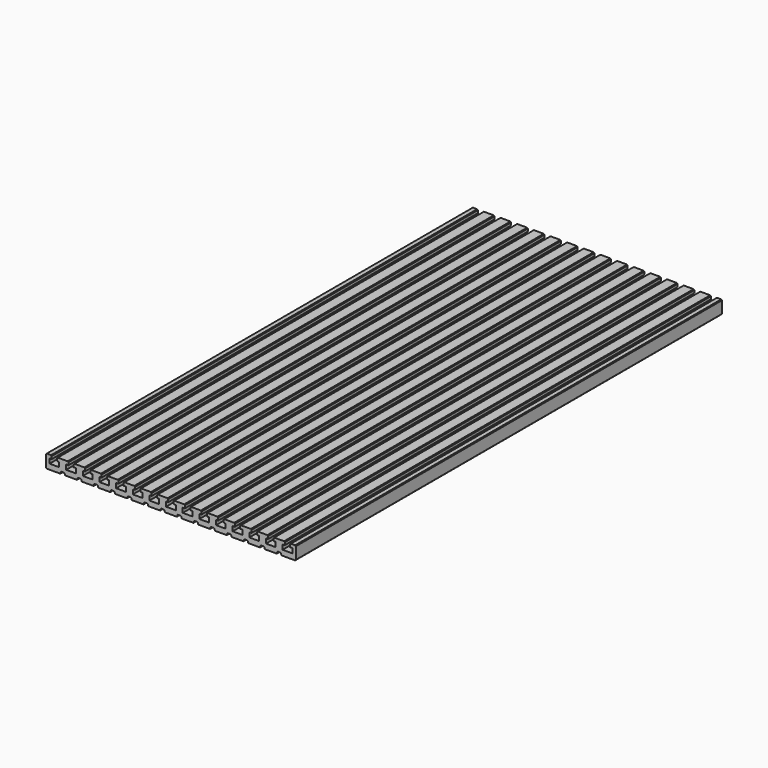
from build123d import *

# Parameters (mm, degrees)
F1_DEPTH = 800


# Not quite as in the source:
# - ends of sketch curves that miss each other by under 0.0002 mm in the source are joined


with BuildPart() as f1:
    # F0 (on Front) → F1 (new body)
    with BuildSketch(Plane.XZ):
        with BuildLine():
            Line((-187.5, -9), (-186.5, -10))
            Line((-186.5, -10), (-166.040705, -10))
            ThreePointArc((-166.040705, -10), (-165.9393586848, -9.787513692), (-165.8725056652, -9.5617878587))
            Line((-165.8725056652, -9.5617878587), (-165.527495, -7.938212))
            ThreePointArc((-165.527495, -7.938212), (-165.0042691575, -7.0843066242), (-164.060257, -6.75))
            Line((-164.060257, -6.75), (-160.939744, -6.75))
            ThreePointArc((-160.939744, -6.75), (-159.9957317617, -7.0843066896), (-159.4725056652, -7.9382121413))
            Line((-159.4725056652, -7.9382121413), (-159.127495, -9.561788))
            ThreePointArc((-159.127495, -9.561788), (-159.0606421883, -9.7875140224), (-158.9592950793, -10.0000000458))
            Line((-158.9592950793, -10.0000000458), (-141.040705, -10))
            ThreePointArc((-141.040705, -10), (-140.9393586848, -9.787513692), (-140.8725056652, -9.5617878587))
            Line((-140.8725056652, -9.5617878587), (-140.527495, -7.938212))
            ThreePointArc((-140.527495, -7.938212), (-140.0042691575, -7.0843066242), (-139.060257, -6.75))
            Line((-139.060257, -6.75), (-135.939744, -6.75))
            ThreePointArc((-135.939744, -6.75), (-134.9957317617, -7.0843066896), (-134.4725056652, -7.9382121413))
            Line((-134.4725056652, -7.9382121413), (-134.127495, -9.561788))
            ThreePointArc((-134.127495, -9.561788), (-134.0606421883, -9.7875140224), (-133.9592950793, -10.0000000458))
            Line((-133.9592950793, -10.0000000458), (-116.040705, -10))
            ThreePointArc((-116.040705, -10), (-115.9393586848, -9.787513692), (-115.8725056652, -9.5617878587))
            Line((-115.8725056652, -9.5617878587), (-115.527495, -7.938212))
            ThreePointArc((-115.527495, -7.938212), (-115.0042691575, -7.0843066242), (-114.060257, -6.75))
            Line((-114.060257, -6.75), (-110.939744, -6.75))
            ThreePointArc((-110.939744, -6.75), (-109.9957317617, -7.0843066896), (-109.4725056652, -7.9382121413))
            Line((-109.4725056652, -7.9382121413), (-109.127495, -9.561788))
            ThreePointArc((-109.127495, -9.561788), (-109.0606421883, -9.7875140224), (-108.9592950793, -10.0000000458))
            Line((-108.9592950793, -10.0000000458), (-91.040705, -10))
            ThreePointArc((-91.040705, -10), (-90.9393586848, -9.787513692), (-90.8725056652, -9.5617878587))
            Line((-90.8725056652, -9.5617878587), (-90.527495, -7.938212))
            ThreePointArc((-90.527495, -7.938212), (-90.0042691575, -7.0843066242), (-89.060257, -6.75))
            Line((-89.060257, -6.75), (-85.939744, -6.75))
            ThreePointArc((-85.939744, -6.75), (-84.9957317617, -7.0843066896), (-84.4725056652, -7.9382121413))
            Line((-84.4725056652, -7.9382121413), (-84.127495, -9.561788))
            ThreePointArc((-84.127495, -9.561788), (-84.0606421883, -9.7875140224), (-83.9592950793, -10.0000000458))
            Line((-83.9592950793, -10.0000000458), (-66.040705, -10))
            ThreePointArc((-66.040705, -10), (-65.9393586848, -9.787513692), (-65.8725056652, -9.5617878587))
            Line((-65.8725056652, -9.5617878587), (-65.527495, -7.938212))
            ThreePointArc((-65.527495, -7.938212), (-65.0042691575, -7.0843066242), (-64.060257, -6.75))
            Line((-64.060257, -6.75), (-60.939744, -6.75))
            ThreePointArc((-60.939744, -6.75), (-59.9957317617, -7.0843066896), (-59.4725056652, -7.9382121413))
            Line((-59.4725056652, -7.9382121413), (-59.127495, -9.561788))
            ThreePointArc((-59.127495, -9.561788), (-59.0606421883, -9.7875140224), (-58.9592950793, -10.0000000458))
            Line((-58.9592950793, -10.0000000458), (-41.040705, -10))
            ThreePointArc((-41.040705, -10), (-40.9393586848, -9.787513692), (-40.8725056652, -9.5617878587))
            Line((-40.8725056652, -9.5617878587), (-40.527495, -7.938212))
            ThreePointArc((-40.527495, -7.938212), (-40.0042691575, -7.0843066242), (-39.060257, -6.75))
            Line((-39.060257, -6.75), (-35.939744, -6.75))
            ThreePointArc((-35.939744, -6.75), (-34.9957317617, -7.0843066896), (-34.4725056652, -7.9382121413))
            Line((-34.4725056652, -7.9382121413), (-34.127495, -9.561788))
            ThreePointArc((-34.127495, -9.561788), (-34.0606421883, -9.7875140224), (-33.9592950793, -10.0000000458))
            Line((-33.9592950793, -10.0000000458), (-16.040705, -10))
            ThreePointArc((-16.040705, -10), (-15.9393586848, -9.787513692), (-15.8725056652, -9.5617878587))
            Line((-15.8725056652, -9.5617878587), (-15.527495, -7.938212))
            ThreePointArc((-15.527495, -7.938212), (-15.0042691575, -7.0843066242), (-14.060257, -6.75))
            Line((-14.060257, -6.75), (-10.939744, -6.75))
            ThreePointArc((-10.939744, -6.75), (-9.9957317617, -7.0843066896), (-9.4725056652, -7.9382121413))
            Line((-9.4725056652, -7.9382121413), (-9.127495, -9.561788))
            ThreePointArc((-9.127495, -9.561788), (-9.0606421883, -9.7875140224), (-8.9592950793, -10.0000000458))
            Line((-8.9592950793, -10.0000000458), (8.959295, -10))
            ThreePointArc((8.959295, -10), (9.0606413152, -9.787513692), (9.1274943348, -9.5617878587))
            Line((9.1274943348, -9.5617878587), (9.472505, -7.938212))
            ThreePointArc((9.472505, -7.938212), (9.9957308425, -7.0843066242), (10.939743, -6.75))
            Line((10.939743, -6.75), (14.060256, -6.75))
            ThreePointArc((14.060256, -6.75), (15.0042682383, -7.0843066896), (15.5274943348, -7.9382121413))
            Line((15.5274943348, -7.9382121413), (15.872505, -9.561788))
            ThreePointArc((15.872505, -9.561788), (15.9393578117, -9.7875140224), (16.0407049207, -10.0000000458))
            Line((16.0407049207, -10.0000000458), (33.959295, -10))
            ThreePointArc((33.959295, -10), (34.0606413152, -9.787513692), (34.1274943348, -9.5617878587))
            Line((34.1274943348, -9.5617878587), (34.472505, -7.938212))
            ThreePointArc((34.472505, -7.938212), (34.9957308425, -7.0843066242), (35.939743, -6.75))
            Line((35.939743, -6.75), (39.060256, -6.75))
            ThreePointArc((39.060256, -6.75), (40.0042682383, -7.0843066896), (40.5274943348, -7.9382121413))
            Line((40.5274943348, -7.9382121413), (40.872505, -9.561788))
            ThreePointArc((40.872505, -9.561788), (40.9393578117, -9.7875140224), (41.0407049207, -10.0000000458))
            Line((41.0407049207, -10.0000000458), (58.959295, -10))
            ThreePointArc((58.959295, -10), (59.0606413152, -9.787513692), (59.1274943348, -9.5617878587))
            Line((59.1274943348, -9.5617878587), (59.472505, -7.938212))
            ThreePointArc((59.472505, -7.938212), (59.9957308425, -7.0843066242), (60.939743, -6.75))
            Line((60.939743, -6.75), (64.060256, -6.75))
            ThreePointArc((64.060256, -6.75), (65.0042682383, -7.0843066896), (65.5274943348, -7.9382121413))
            Line((65.5274943348, -7.9382121413), (65.872505, -9.561788))
            ThreePointArc((65.872505, -9.561788), (65.9393578117, -9.7875140224), (66.0407049207, -10.0000000458))
            Line((66.0407049207, -10.0000000458), (83.959295, -10))
            ThreePointArc((83.959295, -10), (84.0606413152, -9.787513692), (84.1274943348, -9.5617878587))
            Line((84.1274943348, -9.5617878587), (84.472505, -7.938212))
            ThreePointArc((84.472505, -7.938212), (84.9957308425, -7.0843066242), (85.939743, -6.75))
            Line((85.939743, -6.75), (89.060256, -6.75))
            ThreePointArc((89.060256, -6.75), (90.0042682383, -7.0843066896), (90.5274943348, -7.9382121413))
            Line((90.5274943348, -7.9382121413), (90.872505, -9.561788))
            ThreePointArc((90.872505, -9.561788), (90.9393578117, -9.7875140224), (91.0407049207, -10.0000000458))
            Line((91.0407049207, -10.0000000458), (108.959295, -10))
            ThreePointArc((108.959295, -10), (109.0606413152, -9.787513692), (109.1274943348, -9.5617878587))
            Line((109.1274943348, -9.5617878587), (109.472505, -7.938212))
            ThreePointArc((109.472505, -7.938212), (109.9957308425, -7.0843066242), (110.939743, -6.75))
            Line((110.939743, -6.75), (114.060256, -6.75))
            ThreePointArc((114.060256, -6.75), (115.0042682383, -7.0843066896), (115.5274943348, -7.9382121413))
            Line((115.5274943348, -7.9382121413), (115.872505, -9.561788))
            ThreePointArc((115.872505, -9.561788), (115.9393578117, -9.7875140224), (116.0407049207, -10.0000000458))
            Line((116.0407049207, -10.0000000458), (133.959295, -10))
            ThreePointArc((133.959295, -10), (134.0606413152, -9.787513692), (134.1274943348, -9.5617878587))
            Line((134.1274943348, -9.5617878587), (134.472505, -7.938212))
            ThreePointArc((134.472505, -7.938212), (134.9957308425, -7.0843066242), (135.939743, -6.75))
            Line((135.939743, -6.75), (139.060256, -6.75))
            ThreePointArc((139.060256, -6.75), (140.0042682383, -7.0843066896), (140.5274943348, -7.9382121413))
            Line((140.5274943348, -7.9382121413), (140.872505, -9.561788))
            ThreePointArc((140.872505, -9.561788), (140.9393578117, -9.7875140224), (141.0407049207, -10.0000000458))
            Line((141.0407049207, -10.0000000458), (158.959295, -10))
            ThreePointArc((158.959295, -10), (159.0606413152, -9.787513692), (159.1274943348, -9.5617878587))
            Line((159.1274943348, -9.5617878587), (159.472505, -7.938212))
            ThreePointArc((159.472505, -7.938212), (159.9957308425, -7.0843066242), (160.939743, -6.75))
            Line((160.939743, -6.75), (164.060256, -6.75))
            ThreePointArc((164.060256, -6.75), (165.0042682383, -7.0843066896), (165.5274943348, -7.9382121413))
            Line((165.5274943348, -7.9382121413), (165.872505, -9.561788))
            ThreePointArc((165.872505, -9.561788), (165.9393578117, -9.7875140224), (166.0407049207, -10.0000000458))
            Line((166.0407049207, -10.0000000458), (186.5, -10))
            Line((186.5, -10), (187.5, -9))
            Line((187.5, -9), (187.5, 9))
            Line((187.5, 9), (186.5, 10))
            Line((186.5, 10), (180.05, 10))
            Line((180.05, 10), (179.05, 9))
            Line((179.05, 9), (179.05, 5))
            Line((179.05, 5), (182.25, 5))
            Line((182.25, 5), (182.25, -2))
            Line((182.25, -2), (167.75, -2))
            Line((167.75, -2), (167.75, 5))
            Line((167.75, 5), (170.95, 5))
            Line((170.95, 5), (170.95, 9))
            Line((170.95, 9), (169.95, 10))
            Line((169.95, 10), (155.05, 10))
            Line((155.05, 10), (154.05, 9))
            Line((154.05, 9), (154.05, 5))
            Line((154.05, 5), (157.25, 5))
            Line((157.25, 5), (157.25, -2))
            Line((157.25, -2), (142.75, -2))
            Line((142.75, -2), (142.75, 5))
            Line((142.75, 5), (145.95, 5))
            Line((145.95, 5), (145.95, 9))
            Line((145.95, 9), (144.95, 10))
            Line((144.95, 10), (130.05, 10))
            Line((130.05, 10), (129.05, 9))
            Line((129.05, 9), (129.05, 5))
            Line((129.05, 5), (132.25, 5))
            Line((132.25, 5), (132.25, -2))
            Line((132.25, -2), (117.75, -2))
            Line((117.75, -2), (117.75, 5))
            Line((117.75, 5), (120.95, 5))
            Line((120.95, 5), (120.95, 9))
            Line((120.95, 9), (119.95, 10))
            Line((119.95, 10), (105.05, 10))
            Line((105.05, 10), (104.05, 9))
            Line((104.05, 9), (104.05, 5))
            Line((104.05, 5), (107.25, 5))
            Line((107.25, 5), (107.25, -2))
            Line((107.25, -2), (92.75, -2))
            Line((92.75, -2), (92.75, 5))
            Line((92.75, 5), (95.95, 5))
            Line((95.95, 5), (95.95, 9))
            Line((95.95, 9), (94.95, 10))
            Line((94.95, 10), (80.05, 10))
            Line((80.05, 10), (79.05, 9))
            Line((79.05, 9), (79.05, 5))
            Line((79.05, 5), (82.25, 5))
            Line((82.25, 5), (82.25, -2))
            Line((82.25, -2), (67.75, -2))
            Line((67.75, -2), (67.75, 5))
            Line((67.75, 5), (70.95, 5))
            Line((70.95, 5), (70.95, 9))
            Line((70.95, 9), (69.95, 10))
            Line((69.95, 10), (55.05, 10))
            Line((55.05, 10), (54.05, 9))
            Line((54.05, 9), (54.05, 5))
            Line((54.05, 5), (57.25, 5))
            Line((57.25, 5), (57.25, -2))
            Line((57.25, -2), (42.75, -2))
            Line((42.75, -2), (42.75, 5))
            Line((42.75, 5), (45.95, 5))
            Line((45.95, 5), (45.95, 9))
            Line((45.95, 9), (44.95, 10))
            Line((44.95, 10), (30.05, 10))
            Line((30.05, 10), (29.05, 9))
            Line((29.05, 9), (29.05, 5))
            Line((29.05, 5), (32.25, 5))
            Line((32.25, 5), (32.25, -2))
            Line((32.25, -2), (17.75, -2))
            Line((17.75, -2), (17.75, 5))
            Line((17.75, 5), (20.95, 5))
            Line((20.95, 5), (20.95, 9))
            Line((20.95, 9), (19.95, 10))
            Line((19.95, 10), (5.05, 10))
            Line((5.05, 10), (4.05, 9))
            Line((4.05, 9), (4.05, 5))
            Line((4.05, 5), (7.25, 5))
            Line((7.25, 5), (7.25, -2))
            Line((7.25, -2), (-7.25, -2))
            Line((-7.25, -2), (-7.25, 5))
            Line((-7.25, 5), (-4.05, 5))
            Line((-4.05, 5), (-4.05, 9))
            Line((-4.05, 9), (-5.05, 10))
            Line((-5.05, 10), (-19.95, 10))
            Line((-19.95, 10), (-20.95, 9))
            Line((-20.95, 9), (-20.95, 5))
            Line((-20.95, 5), (-17.75, 5))
            Line((-17.75, 5), (-17.75, -2))
            Line((-17.75, -2), (-32.25, -2))
            Line((-32.25, -2), (-32.25, 5))
            Line((-32.25, 5), (-29.05, 5))
            Line((-29.05, 5), (-29.05, 9))
            Line((-29.05, 9), (-30.05, 10))
            Line((-30.05, 10), (-44.95, 10))
            Line((-44.95, 10), (-45.95, 9))
            Line((-45.95, 9), (-45.95, 5))
            Line((-45.95, 5), (-42.75, 5))
            Line((-42.75, 5), (-42.75, -2))
            Line((-42.75, -2), (-57.25, -2))
            Line((-57.25, -2), (-57.25, 5))
            Line((-57.25, 5), (-54.05, 5))
            Line((-54.05, 5), (-54.05, 9))
            Line((-54.05, 9), (-55.05, 10))
            Line((-55.05, 10), (-69.95, 10))
            Line((-69.95, 10), (-70.95, 9))
            Line((-70.95, 9), (-70.95, 5))
            Line((-70.95, 5), (-67.75, 5))
            Line((-67.75, 5), (-67.75, -2))
            Line((-67.75, -2), (-82.25, -2))
            Line((-82.25, -2), (-82.25, 5))
            Line((-82.25, 5), (-79.05, 5))
            Line((-79.05, 5), (-79.05, 9))
            Line((-79.05, 9), (-80.05, 10))
            Line((-80.05, 10), (-94.95, 10))
            Line((-94.95, 10), (-95.95, 9))
            Line((-95.95, 9), (-95.95, 5))
            Line((-95.95, 5), (-92.75, 5))
            Line((-92.75, 5), (-92.75, -2))
            Line((-92.75, -2), (-107.25, -2))
            Line((-107.25, -2), (-107.25, 5))
            Line((-107.25, 5), (-104.05, 5))
            Line((-104.05, 5), (-104.05, 9))
            Line((-104.05, 9), (-105.05, 10))
            Line((-105.05, 10), (-119.95, 10))
            Line((-119.95, 10), (-120.95, 9))
            Line((-120.95, 9), (-120.95, 5))
            Line((-120.95, 5), (-117.75, 5))
            Line((-117.75, 5), (-117.75, -2))
            Line((-117.75, -2), (-132.25, -2))
            Line((-132.25, -2), (-132.25, 5))
            Line((-132.25, 5), (-129.05, 5))
            Line((-129.05, 5), (-129.05, 9))
            Line((-129.05, 9), (-130.05, 10))
            Line((-130.05, 10), (-144.95, 10))
            Line((-144.95, 10), (-145.95, 9))
            Line((-145.95, 9), (-145.95, 5))
            Line((-145.95, 5), (-142.75, 5))
            Line((-142.75, 5), (-142.75, -2))
            Line((-142.75, -2), (-157.25, -2))
            Line((-157.25, -2), (-157.25, 5))
            Line((-157.25, 5), (-154.05, 5))
            Line((-154.05, 5), (-154.05, 9))
            Line((-154.05, 9), (-155.05, 10))
            Line((-155.05, 10), (-169.95, 10))
            Line((-169.95, 10), (-170.95, 9))
            Line((-170.95, 9), (-170.95, 5))
            Line((-170.95, 5), (-167.75, 5))
            Line((-167.75, 5), (-167.75, -2))
            Line((-167.75, -2), (-182.25, -2))
            Line((-182.25, -2), (-182.25, 5))
            Line((-182.25, 5), (-179.05, 5))
            Line((-179.05, 5), (-179.05, 9))
            Line((-179.05, 9), (-180.05, 10))
            Line((-180.05, 10), (-186.5, 10))
            Line((-186.5, 10), (-187.5, 9))
            Line((-187.5, 9), (-187.5, -9))
        make_face()
    extrude(amount=F1_DEPTH)


solid = f1.part
